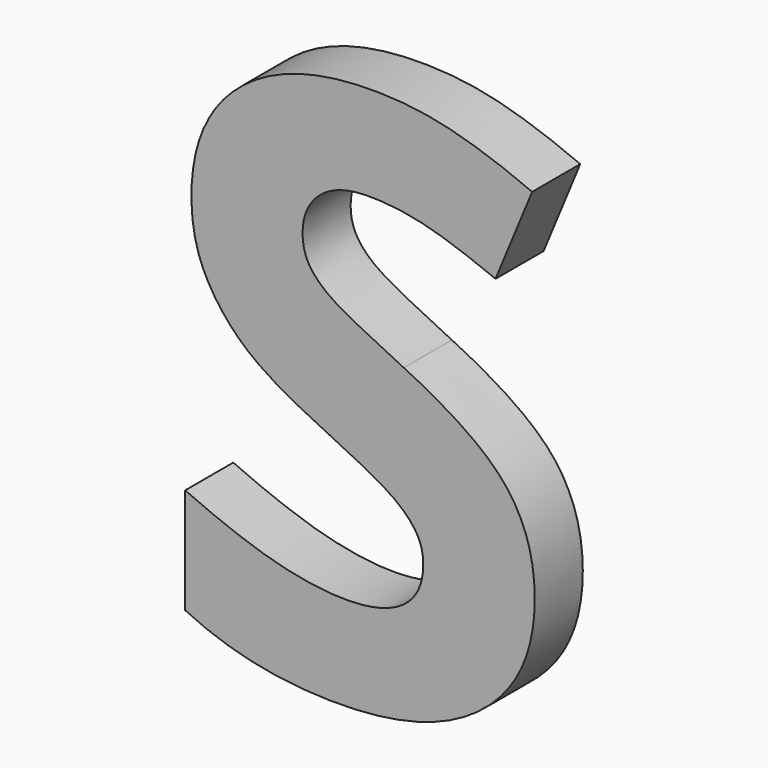
from build123d import *

# Parameters (mm, degrees)
F0_TEXT_SIZE = 62.5
F1_DEPTH     = 5


# Not quite as in the source:
# - Text() gives the source's letters only with a copy of the font that has no kerning and outlines rounded to 1/6400 em; it was checked with that copy


with BuildPart() as f1:
    # F0 (on Front) → F1 (new body)
    with BuildSketch(Plane.XZ):
        with Locations((-58.3527986304, 11.7757008236)):
            Text('S', F0_TEXT_SIZE, font='Open Sans', font_style=FontStyle.BOLD, text_align=(TextAlign.LEFT, TextAlign.BOTTOM))
    extrude(amount=F1_DEPTH)


solid = f1.part
